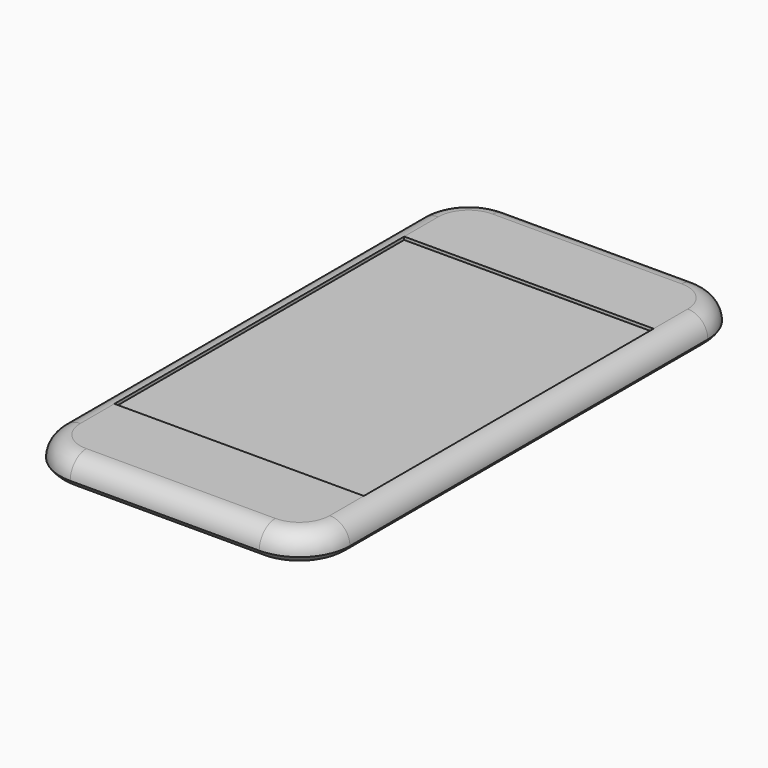
from build123d import *

# Parameters (mm, degrees)
F1_DEPTH     = 7.4836481363
F2_R         = 5.08
F3_T1_DEPTH  = 47.6248391628
F3_T3_DEPTH  = 112.7664723158
F3_T6_ANGLE  = 90
F3_T8_ANGLE  = 90
F3_T10_ANGLE = 90
F3_T12_ANGLE = 90
F4_W         = 62.8648391628
F4_H         = 91.2811607122
F5_DEPTH     = 0.7581766695


# Not quite as in the source:
# - a fillet or chamfer that OpenCascade refuses, or shapes differently, is made with other operations: its cross-section is extruded or revolved along the edge and cut away or added


with BuildPart() as f1:
    # F0 (on Top) → F1 (new body)
    with BuildSketch(Plane.XY):
        with BuildLine():
            ThreePointArc((36.5124195814, 56.3832361579), (32.7926757025, 65.363492279), (23.8124195814, 69.0832361579))
            Line((23.8124195814, 69.0832361579), (-23.8124195814, 69.0832361579))
            ThreePointArc((-23.8124195814, 69.0832361579), (-32.7926757025, 65.363492279), (-36.5124195814, 56.3832361579))
            Line((-36.5124195814, 56.3832361579), (-36.5124195814, -56.3832361579))
            ThreePointArc((-36.5124195814, -56.3832361579), (-32.7926757025, -65.363492279), (-23.8124195814, -69.0832361579))
            Line((-23.8124195814, -69.0832361579), (23.8124195814, -69.0832361579))
            ThreePointArc((23.8124195814, -69.0832361579), (32.7926757025, -65.363492279), (36.5124195814, -56.3832361579))
            Line((36.5124195814, -56.3832361579), (36.5124195814, 56.3832361579))
        make_face()
    extrude(amount=F1_DEPTH)

    # F2
    f2_edges = [f1.edges().sort_by_distance(p)[0] for p in [
        (0, -69.083236, 7.483648),
    ]]
    fillet(f2_edges, radius=F2_R)

    # F3: fillet of radius 5.08 on 1 edges, made by hand

    # F3_s2 → F3_t1 (cut)
    with BuildSketch(Plane.YZ.offset(-23.8124195814)):
        with BuildLine():
            ThreePointArc((-64.7654194988, 0), (-67.2363032003, 0.6414040808), (-69.0832361579, 2.4036481363))
            Line((-69.0832361579, 2.4036481363), (-69.0832361579, 0))
            Line((-69.0832361579, 0), (-64.7654194988, 0))
        make_face()
        with BuildLine():
            ThreePointArc((64.7654194988, 0), (67.2363032003, 0.6414040808), (69.0832361579, 2.4036481363))
            Line((69.0832361579, 2.4036481363), (69.0832361579, 0))
            Line((69.0832361579, 0), (64.7654194988, 0))
        make_face()
    extrude(amount=F3_T1_DEPTH, mode=Mode.SUBTRACT)

    # F3_s4 → F3_t3 (cut)
    with BuildSketch(Plane.XZ.offset(-56.3832361579)):
        with BuildLine():
            ThreePointArc((36.5124195814, 2.4036481363), (34.6654866238, 0.6414040808), (32.1946029223, 0))
            Line((32.1946029223, 0), (36.5124195814, 0))
            Line((36.5124195814, 0), (36.5124195814, 2.4036481363))
        make_face()
        with BuildLine():
            ThreePointArc((-32.1946029223, 0), (-34.6654866238, 0.6414040808), (-36.5124195814, 2.4036481363))
            Line((-36.5124195814, 2.4036481363), (-36.5124195814, 0))
            Line((-36.5124195814, 0), (-32.1946029223, 0))
        make_face()
    extrude(amount=F3_T3_DEPTH, mode=Mode.SUBTRACT)

    # F3_s5 → F3_t6 (revolve, cut)
    with BuildSketch(Plane.XZ.offset(56.3832361579)):
        with BuildLine():
            ThreePointArc((-32.1946029223, 0), (-34.6654866238, 0.6414040808), (-36.5124195814, 2.4036481363))
            Line((-36.5124195814, 2.4036481363), (-36.5124195814, 0))
            Line((-36.5124195814, 0), (-32.1946029223, 0))
        make_face()
    revolve(axis=Axis((-23.8124195814, -56.3832361579, 0), (0, 0, 1)), revolution_arc=F3_T6_ANGLE, mode=Mode.SUBTRACT)

    # F3_s7 → F3_t8 (revolve, cut)
    with BuildSketch(Plane.YZ.offset(23.8124195814)):
        with BuildLine():
            ThreePointArc((-64.7654194988, 0), (-67.2363032003, 0.6414040808), (-69.0832361579, 2.4036481363))
            Line((-69.0832361579, 2.4036481363), (-69.0832361579, 0))
            Line((-69.0832361579, 0), (-64.7654194988, 0))
        make_face()
    revolve(axis=Axis((23.8124195814, -56.3832361579, 0), (0, 0, 1)), revolution_arc=F3_T8_ANGLE, mode=Mode.SUBTRACT)

    # F3_s9 → F3_t10 (revolve, cut)
    with BuildSketch(Plane.XZ.offset(-56.3832361579)):
        with BuildLine():
            ThreePointArc((36.5124195814, 2.4036481363), (34.6654866238, 0.6414040808), (32.1946029223, 0))
            Line((32.1946029223, 0), (36.5124195814, 0))
            Line((36.5124195814, 0), (36.5124195814, 2.4036481363))
        make_face()
    revolve(axis=Axis((23.8124195814, 56.3832361579, 0), (0, 0, 1)), revolution_arc=F3_T10_ANGLE, mode=Mode.SUBTRACT)

    # F3_s11 → F3_t12 (revolve, cut)
    with BuildSketch(Plane.YZ.offset(-23.8124195814)):
        with BuildLine():
            ThreePointArc((64.7654194988, 0), (67.2363032003, 0.6414040808), (69.0832361579, 2.4036481363))
            Line((69.0832361579, 2.4036481363), (69.0832361579, 0))
            Line((69.0832361579, 0), (64.7654194988, 0))
        make_face()
    revolve(axis=Axis((-23.8124195814, 56.3832361579, 0), (0, 0, 1)), revolution_arc=F3_T12_ANGLE, mode=Mode.SUBTRACT)

    # F4 (on face) → F5 (cut)
    with BuildSketch(Plane.XY.offset(7.4836481363)):
        Rectangle(F4_W, F4_H)
    extrude(amount=-F5_DEPTH, mode=Mode.SUBTRACT)


solid = f1.part
